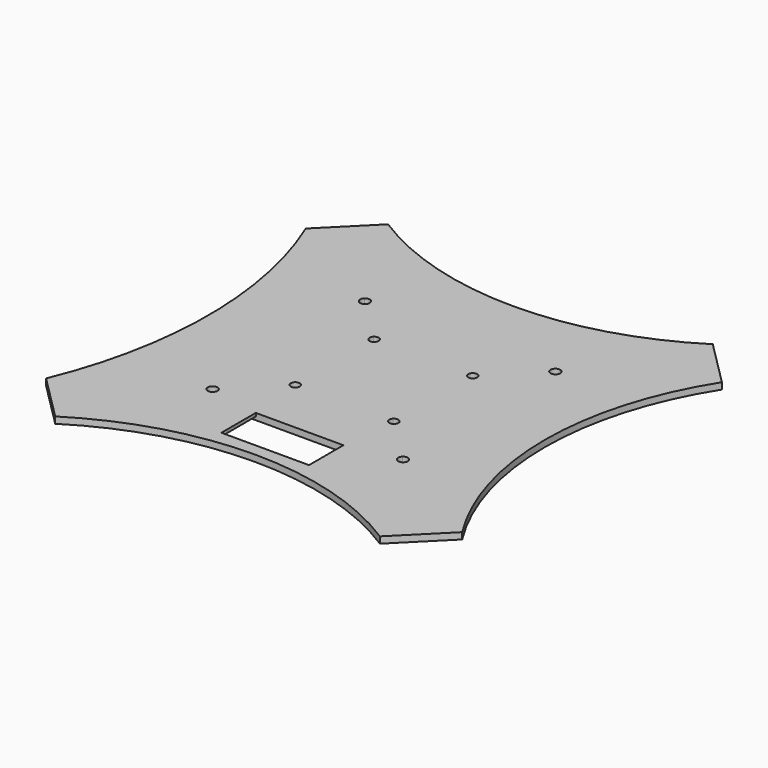
from build123d import *

# Parameters (mm, degrees)
F0_W     = 4
F0_H     = 13.3
F1_DEPTH = 2
F2_DEPTH = 3
F0_W_2   = 27.1
F3_DEPTH = 1


with BuildPart() as f1:
    # F0 (on Top) → F1 (new body)
    with BuildSketch(Plane.XY):
        with BuildLine():
            Line((-30.504587, 30.504587), (-57.275649, 57.275649))
            Line((-57.275649, 57.275649), (-64.346717, 50.204581))
            ThreePointArc((-64.346717, 50.204581), (-54.365208, 0), (-64.346717, -50.204581))
            Line((-64.346717, -50.204581), (-57.275649, -57.275649))
            Line((-57.275649, -57.275649), (-30.504587, -30.504587))
            ThreePointArc((-30.504587, -30.504587), (-30.504587, -28.383266), (-28.383266, -28.383266))
            Line((-28.383266, -28.383266), (-17.017767, -17.017767))
            ThreePointArc((-17.017767, -17.017767), (-17.017767, -13.482233), (-13.482233, -13.482233))
            Line((-13.482233, -13.482233), (0, 0))
            Line((0, 0), (-13.482233, 13.482233))
            ThreePointArc((-13.482233, 13.482233), (-17.017767, 13.482233), (-17.017767, 17.017767))
            Line((-17.017767, 17.017767), (-28.383266, 28.383266))
            ThreePointArc((-28.383266, 28.383266), (-30.504587, 28.383266), (-30.504587, 30.504587))
        make_face()
        with BuildLine():
            Line((-30.504587, -30.504587), (-57.275649, -57.275649))
            Line((-57.275649, -57.275649), (-50.204581, -64.346717))
            ThreePointArc((-50.204581, -64.346717), (0, -49.764969), (50.204581, -64.346717))
            Line((50.204581, -64.346717), (57.275649, -57.275649))
            Line((57.275649, -57.275649), (30.504587, -30.504587))
            ThreePointArc((30.504587, -30.504587), (28.383266, -30.504587), (28.383266, -28.383266))
            Line((28.383266, -28.383266), (17.017767, -17.017767))
            ThreePointArc((17.017767, -17.017767), (13.482233, -17.017767), (13.482233, -13.482233))
            Line((13.482233, -13.482233), (0, 0))
            Line((0, 0), (-13.482233, -13.482233))
            ThreePointArc((-13.482233, -13.482233), (-12.940301, -14.293291), (-12.75, -15.25))
            ThreePointArc((-12.75, -15.25), (-14.293291, -17.559699), (-17.017767, -17.017767))
            Line((-17.017767, -17.017767), (-28.383266, -28.383266))
            ThreePointArc((-28.383266, -28.383266), (-28.058107, -28.869901), (-27.943926, -29.443926))
            ThreePointArc((-27.943926, -29.443926), (-28.869901, -30.829746), (-30.504587, -30.504587))
        make_face()
        Polygon((17.55, -32.633641), (17.55, -45.933641), (13.55, -45.933641), (-13.55, -45.933641), (-17.55, -45.933641), (-17.55, -32.633641), (-13.55, -32.633641), (13.55, -32.633641), align=None, mode=Mode.SUBTRACT)
        with BuildLine():
            ThreePointArc((50.204581, 64.346717), (0, 49.764969), (-50.204581, 64.346717))
            Line((-50.204581, 64.346717), (-57.275649, 57.275649))
            Line((-57.275649, 57.275649), (-30.504587, 30.504587))
            ThreePointArc((-30.504587, 30.504587), (-28.869901, 30.829746), (-27.943926, 29.443926))
            ThreePointArc((-27.943926, 29.443926), (-28.058107, 28.869901), (-28.383266, 28.383266))
            Line((-28.383266, 28.383266), (-17.017767, 17.017767))
            ThreePointArc((-17.017767, 17.017767), (-14.293291, 17.559699), (-12.75, 15.25))
            ThreePointArc((-12.75, 15.25), (-12.940301, 14.293291), (-13.482233, 13.482233))
            Line((-13.482233, 13.482233), (0, 0))
            Line((0, 0), (13.482233, 13.482233))
            ThreePointArc((13.482233, 13.482233), (13.482233, 17.017767), (17.017767, 17.017767))
            Line((17.017767, 17.017767), (28.383266, 28.383266))
            ThreePointArc((28.383266, 28.383266), (28.383266, 30.504587), (30.504587, 30.504587))
            Line((30.504587, 30.504587), (57.275649, 57.275649))
            Line((57.275649, 57.275649), (50.204581, 64.346717))
        make_face()
        with BuildLine():
            Line((64.346717, 50.204581), (57.275649, 57.275649))
            Line((57.275649, 57.275649), (30.504587, 30.504587))
            ThreePointArc((30.504587, 30.504587), (30.829746, 30.017952), (30.943926, 29.443926))
            ThreePointArc((30.943926, 29.443926), (30.017952, 28.058107), (28.383266, 28.383266))
            Line((28.383266, 28.383266), (17.017767, 17.017767))
            ThreePointArc((17.017767, 17.017767), (17.559699, 16.206709), (17.75, 15.25))
            ThreePointArc((17.75, 15.25), (16.206709, 12.940301), (13.482233, 13.482233))
            Line((13.482233, 13.482233), (0, 0))
            Line((0, 0), (13.482233, -13.482233))
            ThreePointArc((13.482233, -13.482233), (16.206709, -12.940301), (17.75, -15.25))
            ThreePointArc((17.75, -15.25), (17.559699, -16.206709), (17.017767, -17.017767))
            Line((17.017767, -17.017767), (28.383266, -28.383266))
            ThreePointArc((28.383266, -28.383266), (30.017952, -28.058107), (30.943926, -29.443926))
            ThreePointArc((30.943926, -29.443926), (30.829746, -30.017952), (30.504587, -30.504587))
            Line((30.504587, -30.504587), (57.275649, -57.275649))
            Line((57.275649, -57.275649), (64.346717, -50.204581))
            ThreePointArc((64.346717, -50.204581), (49.764969, 0), (64.346717, 50.204581))
        make_face()
        with Locations((15.55, -39.283641)):
            Rectangle(F0_W, F0_H)
        with Locations((-15.55, -39.283641)):
            Rectangle(F0_W, F0_H)
        with BuildLine():
            Line((-16.239949, 16.239949), (-17.017767, 17.017767))
            ThreePointArc((-17.017767, 17.017767), (-17.017767, 13.482233), (-13.482233, 13.482233))
            Line((-13.482233, 13.482233), (-14.260051, 14.260051))
            ThreePointArc((-14.260051, 14.260051), (-16.239949, 14.260051), (-16.239949, 16.239949))
        make_face()
        with BuildLine():
            ThreePointArc((-12.75, 15.25), (-14.293291, 17.559699), (-17.017767, 17.017767))
            Line((-17.017767, 17.017767), (-16.239949, 16.239949))
            ThreePointArc((-16.239949, 16.239949), (-14.714243, 16.543431), (-13.85, 15.25))
            ThreePointArc((-13.85, 15.25), (-13.956569, 14.714243), (-14.260051, 14.260051))
            Line((-14.260051, 14.260051), (-13.482233, 13.482233))
            ThreePointArc((-13.482233, 13.482233), (-12.940301, 14.293291), (-12.75, 15.25))
        make_face()
        with BuildLine():
            Line((16.239949, 16.239949), (17.017767, 17.017767))
            ThreePointArc((17.017767, 17.017767), (13.482233, 17.017767), (13.482233, 13.482233))
            Line((13.482233, 13.482233), (14.260051, 14.260051))
            ThreePointArc((14.260051, 14.260051), (14.260051, 16.239949), (16.239949, 16.239949))
        make_face()
        with BuildLine():
            ThreePointArc((17.75, 15.25), (17.559699, 16.206709), (17.017767, 17.017767))
            Line((17.017767, 17.017767), (16.239949, 16.239949))
            ThreePointArc((16.239949, 16.239949), (16.543431, 15.785757), (16.65, 15.25))
            ThreePointArc((16.65, 15.25), (15.785757, 13.956569), (14.260051, 14.260051))
            Line((14.260051, 14.260051), (13.482233, 13.482233))
            ThreePointArc((13.482233, 13.482233), (16.206709, 12.940301), (17.75, 15.25))
        make_face()
        with BuildLine():
            Line((14.260051, -14.260051), (13.482233, -13.482233))
            ThreePointArc((13.482233, -13.482233), (13.482233, -17.017767), (17.017767, -17.017767))
            Line((17.017767, -17.017767), (16.239949, -16.239949))
            ThreePointArc((16.239949, -16.239949), (14.260051, -16.239949), (14.260051, -14.260051))
        make_face()
        with BuildLine():
            ThreePointArc((17.75, -15.25), (16.206709, -12.940301), (13.482233, -13.482233))
            Line((13.482233, -13.482233), (14.260051, -14.260051))
            ThreePointArc((14.260051, -14.260051), (15.785757, -13.956569), (16.65, -15.25))
            ThreePointArc((16.65, -15.25), (16.543431, -15.785757), (16.239949, -16.239949))
            Line((16.239949, -16.239949), (17.017767, -17.017767))
            ThreePointArc((17.017767, -17.017767), (17.559699, -16.206709), (17.75, -15.25))
        make_face()
        with BuildLine():
            ThreePointArc((-13.482233, -13.482233), (-17.017767, -13.482233), (-17.017767, -17.017767))
            Line((-17.017767, -17.017767), (-16.239949, -16.239949))
            ThreePointArc((-16.239949, -16.239949), (-16.239949, -14.260051), (-14.260051, -14.260051))
            Line((-14.260051, -14.260051), (-13.482233, -13.482233))
        make_face()
        with BuildLine():
            Line((-16.239949, -16.239949), (-17.017767, -17.017767))
            ThreePointArc((-17.017767, -17.017767), (-14.293291, -17.559699), (-12.75, -15.25))
            ThreePointArc((-12.75, -15.25), (-12.940301, -14.293291), (-13.482233, -13.482233))
            Line((-13.482233, -13.482233), (-14.260051, -14.260051))
            ThreePointArc((-14.260051, -14.260051), (-13.956569, -14.714243), (-13.85, -15.25))
            ThreePointArc((-13.85, -15.25), (-14.714243, -16.543431), (-16.239949, -16.239949))
        make_face()
    extrude(amount=F1_DEPTH)

    # F0 (on Top) → F2 (join)
    with BuildSketch(Plane.XY):
        with BuildLine():
            Line((-16.239949, 16.239949), (-17.017767, 17.017767))
            ThreePointArc((-17.017767, 17.017767), (-17.017767, 13.482233), (-13.482233, 13.482233))
            Line((-13.482233, 13.482233), (-14.260051, 14.260051))
            ThreePointArc((-14.260051, 14.260051), (-16.239949, 14.260051), (-16.239949, 16.239949))
        make_face()
        with BuildLine():
            ThreePointArc((-12.75, 15.25), (-14.293291, 17.559699), (-17.017767, 17.017767))
            Line((-17.017767, 17.017767), (-16.239949, 16.239949))
            ThreePointArc((-16.239949, 16.239949), (-14.714243, 16.543431), (-13.85, 15.25))
            ThreePointArc((-13.85, 15.25), (-13.956569, 14.714243), (-14.260051, 14.260051))
            Line((-14.260051, 14.260051), (-13.482233, 13.482233))
            ThreePointArc((-13.482233, 13.482233), (-12.940301, 14.293291), (-12.75, 15.25))
        make_face()
        with BuildLine():
            Line((16.239949, 16.239949), (17.017767, 17.017767))
            ThreePointArc((17.017767, 17.017767), (13.482233, 17.017767), (13.482233, 13.482233))
            Line((13.482233, 13.482233), (14.260051, 14.260051))
            ThreePointArc((14.260051, 14.260051), (14.260051, 16.239949), (16.239949, 16.239949))
        make_face()
        with BuildLine():
            ThreePointArc((17.75, 15.25), (17.559699, 16.206709), (17.017767, 17.017767))
            Line((17.017767, 17.017767), (16.239949, 16.239949))
            ThreePointArc((16.239949, 16.239949), (16.543431, 15.785757), (16.65, 15.25))
            ThreePointArc((16.65, 15.25), (15.785757, 13.956569), (14.260051, 14.260051))
            Line((14.260051, 14.260051), (13.482233, 13.482233))
            ThreePointArc((13.482233, 13.482233), (16.206709, 12.940301), (17.75, 15.25))
        make_face()
        with BuildLine():
            ThreePointArc((-13.482233, -13.482233), (-17.017767, -13.482233), (-17.017767, -17.017767))
            Line((-17.017767, -17.017767), (-16.239949, -16.239949))
            ThreePointArc((-16.239949, -16.239949), (-16.239949, -14.260051), (-14.260051, -14.260051))
            Line((-14.260051, -14.260051), (-13.482233, -13.482233))
        make_face()
        with BuildLine():
            Line((-16.239949, -16.239949), (-17.017767, -17.017767))
            ThreePointArc((-17.017767, -17.017767), (-14.293291, -17.559699), (-12.75, -15.25))
            ThreePointArc((-12.75, -15.25), (-12.940301, -14.293291), (-13.482233, -13.482233))
            Line((-13.482233, -13.482233), (-14.260051, -14.260051))
            ThreePointArc((-14.260051, -14.260051), (-13.956569, -14.714243), (-13.85, -15.25))
            ThreePointArc((-13.85, -15.25), (-14.714243, -16.543431), (-16.239949, -16.239949))
        make_face()
        with BuildLine():
            Line((14.260051, -14.260051), (13.482233, -13.482233))
            ThreePointArc((13.482233, -13.482233), (13.482233, -17.017767), (17.017767, -17.017767))
            Line((17.017767, -17.017767), (16.239949, -16.239949))
            ThreePointArc((16.239949, -16.239949), (14.260051, -16.239949), (14.260051, -14.260051))
        make_face()
        with BuildLine():
            ThreePointArc((17.75, -15.25), (16.206709, -12.940301), (13.482233, -13.482233))
            Line((13.482233, -13.482233), (14.260051, -14.260051))
            ThreePointArc((14.260051, -14.260051), (15.785757, -13.956569), (16.65, -15.25))
            ThreePointArc((16.65, -15.25), (16.543431, -15.785757), (16.239949, -16.239949))
            Line((16.239949, -16.239949), (17.017767, -17.017767))
            ThreePointArc((17.017767, -17.017767), (17.559699, -16.206709), (17.75, -15.25))
        make_face()
    extrude(amount=-F2_DEPTH)

    # F0 (on Top) → F3 (cut)
    with BuildSketch(Plane.XY):
        with Locations((15.55, -39.283641)):
            Rectangle(F0_W, F0_H)
        with Locations((0, -39.283641)):
            Rectangle(F0_W_2, F0_H)
        with Locations((-15.55, -39.283641)):
            Rectangle(F0_W, F0_H)
    extrude(amount=F3_DEPTH, mode=Mode.SUBTRACT)


solid = f1.part
